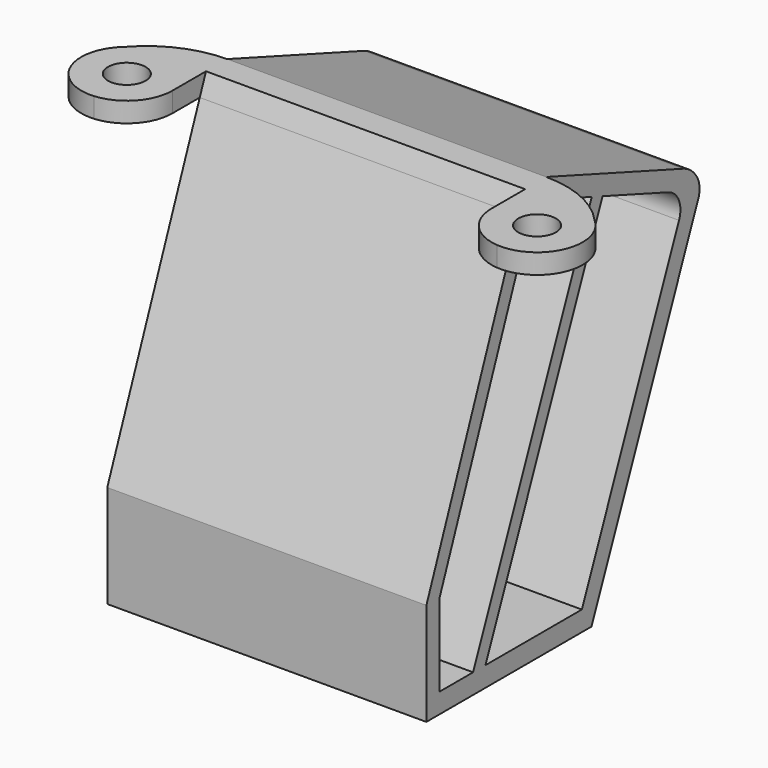
from build123d import *

# Parameters (mm, degrees)
F1_DEPTH   = 28
F2_R       = 1.65
F3_DEPTH   = 1.75
F1_FACE1_W = 28
F1_FACE1_H = 1.75
F4_REACH   = 50.8712690127


with BuildPart() as f1:
    # F0 (on Right) → F1 (new body)
    with BuildSketch(Plane.YZ):
        with BuildLine():
            Line((-3, 35), (0, 35))
            Line((0, 35), (-10.1456508905, 9.0044083693))
            Line((-10.1456508905, 9.0044083693), (-10.1456508905, 0))
            Line((-10.1456508905, 0), (7.9644151033, 0))
            Line((7.9644151033, 0), (19.6633343933, 28.2374824987))
            ThreePointArc((19.6633343933, 28.2374824987), (19.8121032451, 29.121794497), (19.559512125, 29.9822232317))
            ThreePointArc((19.559512125, 29.9822232317), (18.9135949962, 30.766804474), (18.0350819326, 31.2776777068))
            Line((18.0350819326, 31.2776777068), (3, 36.75))
            Line((3, 36.75), (0, 36.75))
            Line((0, 36.75), (-3, 36.75))
            Line((-3, 36.75), (-3, 35))
        make_face()
        with BuildLine():
            Line((-8.6863745263, 9.0319523177), (1.4485264153, 35))
            Line((1.4485264153, 35), (3, 35))
            Line((3, 35), (8.0000780063, 33.1801204367))
            Line((8.0000780063, 33.1801204367), (9.1758168143, 32.7521865073))
            Line((9.1758168143, 32.7521865073), (16.3991077878, 30.1231235995))
            ThreePointArc((16.3991077878, 30.1231235995), (17.5457217574, 29.0491606036), (17.5627670801, 27.4782278969))
            Line((17.5627670801, 27.4782278969), (6.9034435496, 1.75))
            Line((6.9034435496, 1.75), (-3.6685321031, 1.75))
            Line((-3.6685321031, 1.75), (-5.0215659125, 1.75))
            Line((-5.0215659125, 1.75), (-8.6863745263, 1.75))
            Line((-8.6863745263, 1.75), (-8.6863745263, 9.0319523177))
        make_face(mode=Mode.SUBTRACT)
        Polygon((9.1758168143, 32.7521865073), (8.0000780063, 33.1801204367), (-5.0215659125, 1.75), (-3.6685321031, 1.75), align=None)
    extrude(amount=F1_DEPTH)

    # F2 (on face) → F3 (join)
    with BuildSketch(Plane.XY.offset(36.75)):
        with BuildLine():
            Line((0, -3), (0, 3))
            ThreePointArc((0, 3), (-3.6457513111, 2.215250437), (-6.6457513111, 0))
            ThreePointArc((-6.6457513111, 0), (-7.6807421272, -4.5659302006), (-3.673363624, -6.9866412778))
            ThreePointArc((-3.673363624, -6.9866412778), (-1.0583554341, -5.7104846888), (0, -3))
        make_face()
        with Locations((-4, -3)):
            Circle(F2_R, mode=Mode.SUBTRACT)
        with BuildLine():
            ThreePointArc((34.6457513111, 0), (31.6457513111, 2.215250437), (28, 3))
            Line((28, 3), (28, -3))
            ThreePointArc((28, -3), (29.0583554341, -5.7104846888), (31.673363624, -6.9866412778))
            ThreePointArc((31.673363624, -6.9866412778), (35.6807421272, -4.5659302006), (34.6457513111, 0))
        make_face()
        with Locations((32, -3)):
            Circle(F2_R, mode=Mode.SUBTRACT)
    extrude(amount=-F3_DEPTH)

    f4_end = Plane(origin=(14, -5.0728254453, 22.0022041847), x_dir=(0, -0.3635745105, -0.9315651213), z_dir=(0, -0.9315651213, 0.3635745105))
    # F1_face1 (on face) → F4 (cut, up to a plane its end follows)
    with BuildSketch(Plane(origin=(14, -3, 35.875), x_dir=(1, 0, 0), z_dir=(0, -1, 0))):
        Rectangle(F1_FACE1_W, F1_FACE1_H)
    f4_long = extrude(amount=-F4_REACH, mode=Mode.PRIVATE)
    add(split(f4_long, bisect_by=f4_end, keep=Keep.TOP, mode=Mode.PRIVATE), mode=Mode.SUBTRACT)


solid = f1.part
